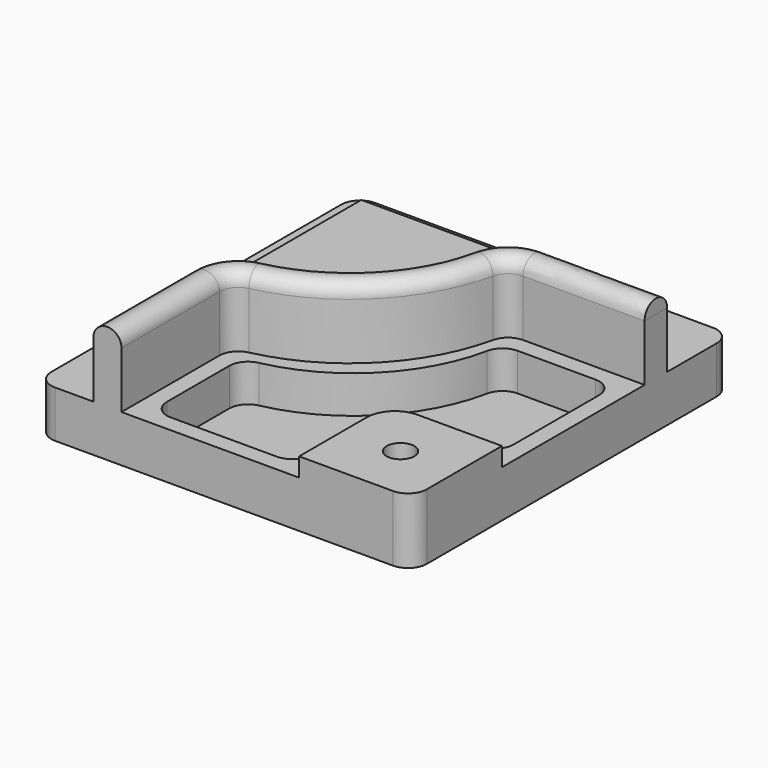
from build123d import *

# Parameters (mm, degrees)
F1_DEPTH        = 35
F2_DEPTH        = 25
F3_DEPTH        = 55
F4_DEPTH        = 25
F5_DEPTH        = 33
F6_DEPTH        = 5
F9_SIZE         = 4.5
F10_D           = 14.75
F10_CBORE_D     = 22.25
F10_CBORE_DEPTH = 14


with BuildPart() as f1:
    # F0 (on Top) → F1 (new body)
    with BuildSketch(Plane.XY):
        with BuildLine():
            Line((100, -96.5), (100, -46.5))
            Line((100, -46.5), (55, -46.5))
            ThreePointArc((55, -46.5), (44.393398, -50.893398), (40, -61.5))
            Line((40, -61.5), (40, -106.5))
            Line((40, -106.5), (90, -106.5))
            ThreePointArc((90, -106.5), (97.071068, -103.571068), (100, -96.5))
        make_face()
    extrude(amount=F1_DEPTH)

    # F0 (on Top) → F2 (join)
    with BuildSketch(Plane.XY):
        with BuildLine():
            Line((100, -46.5), (100, 48.5))
            Line((100, 48.5), (35.260832, 48.5))
            ThreePointArc((35.260832, 48.5), (29.00115, 46.298485), (25.497624, 40.663275))
            ThreePointArc((25.497624, 40.663275), (-0.104824, -5.979511), (-46.775973, -31.53022))
            ThreePointArc((-46.775973, -31.53022), (-52.418539, -35.031816), (-54.623526, -41.295822))
            Line((-54.623526, -41.295822), (-54.623526, -106.5))
            Line((-54.623526, -106.5), (40, -106.5))
            Line((40, -106.5), (40, -61.5))
            ThreePointArc((40, -61.5), (44.393398, -50.893398), (55, -46.5))
            Line((55, -46.5), (100, -46.5))
        make_face()
        with BuildLine():
            Line((31, -62.5), (31, -87.5))
            ThreePointArc((31, -87.5), (28.071068, -94.571068), (21, -97.5))
            Line((21, -97.5), (-35.623526, -97.5))
            ThreePointArc((-35.623526, -97.5), (-42.694594, -94.571068), (-45.623526, -87.5))
            Line((-45.623526, -87.5), (-45.623526, -46.002816))
            ThreePointArc((-45.623526, -46.002816), (-43.385729, -39.698199), (-37.673886, -36.215272))
            ThreePointArc((-37.673886, -36.215272), (6.161704, -12.434582), (29.746581, 31.506672))
            ThreePointArc((29.746581, 31.506672), (33.221258, 37.24812), (39.543175, 39.5))
            Line((39.543175, 39.5), (81, 39.5))
            ThreePointArc((81, 39.5), (88.071068, 36.571068), (91, 29.5))
            Line((91, 29.5), (91, -27.5))
            ThreePointArc((91, -27.5), (88.071068, -34.571068), (81, -37.5))
            Line((81, -37.5), (56, -37.5))
            ThreePointArc((56, -37.5), (38.32233, -44.82233), (31, -62.5))
        make_face(mode=Mode.SUBTRACT)
    extrude(amount=F2_DEPTH)

    # F0 (on Top) → F3 (join)
    with BuildSketch(Plane.XY):
        with BuildLine():
            Line((100, 48.5), (100, 63.5))
            Line((100, 63.5), (35.735586, 63.5))
            ThreePointArc((35.735586, 63.5), (20.232292, 58.112442), (11.41099, 44.27183))
            ThreePointArc((11.41099, 44.27183), (-10.73246, 4.608934), (-50.395356, -17.534515))
            ThreePointArc((-50.395356, -17.534515), (-64.235968, -26.355818), (-69.623526, -41.859112))
            Line((-69.623526, -41.859112), (-69.623526, -106.5))
            Line((-69.623526, -106.5), (-54.623526, -106.5))
            Line((-54.623526, -106.5), (-54.623526, -41.295822))
            ThreePointArc((-54.623526, -41.295822), (-52.418539, -35.031816), (-46.775973, -31.53022))
            ThreePointArc((-46.775973, -31.53022), (-0.104824, -5.979511), (25.497624, 40.663275))
            ThreePointArc((25.497624, 40.663275), (29.00115, 46.298485), (35.260832, 48.5))
            Line((35.260832, 48.5), (100, 48.5))
        make_face()
    extrude(amount=F3_DEPTH)

    # F0 (on Top) → F4 (join)
    with BuildSketch(Plane.XY):
        with BuildLine():
            Line((90, 106.5), (-90, 106.5))
            ThreePointArc((-90, 106.5), (-97.071068, 103.571068), (-100, 96.5))
            Line((-100, 96.5), (-100, -96.5))
            ThreePointArc((-100, -96.5), (-97.071068, -103.571068), (-90, -106.5))
            Line((-90, -106.5), (-69.623526, -106.5))
            Line((-69.623526, -106.5), (-69.623526, -41.859112))
            ThreePointArc((-69.623526, -41.859112), (-64.235968, -26.355818), (-50.395356, -17.534515))
            ThreePointArc((-50.395356, -17.534515), (-10.73246, 4.608934), (11.41099, 44.27183))
            ThreePointArc((11.41099, 44.27183), (20.232292, 58.112442), (35.735586, 63.5))
            Line((35.735586, 63.5), (100, 63.5))
            Line((100, 63.5), (100, 96.5))
            ThreePointArc((100, 96.5), (97.071068, 103.571068), (90, 106.5))
        make_face()
        with BuildLine():
            ThreePointArc((3.895179, 97.5), (-7.793942, 11.173118), (-91, -14.628397))
            Line((-91, -14.628397), (-91, 97.5))
            Line((-91, 97.5), (3.895179, 97.5))
        make_face(mode=Mode.SUBTRACT)
    extrude(amount=F4_DEPTH)

    # F0 (on Top) → F5 (join)
    with BuildSketch(Plane.XY):
        with BuildLine():
            Line((-91, 97.5), (-91, -14.628397))
            ThreePointArc((-91, -14.628397), (-7.793942, 11.173118), (3.895179, 97.5))
            Line((3.895179, 97.5), (-91, 97.5))
        make_face()
    extrude(amount=F5_DEPTH)

    # F0 (on Top) → F6 (join)
    with BuildSketch(Plane.XY):
        with BuildLine():
            ThreePointArc((21, -97.5), (28.071068, -94.571068), (31, -87.5))
            Line((31, -87.5), (31, -62.5))
            ThreePointArc((31, -62.5), (38.32233, -44.82233), (56, -37.5))
            Line((56, -37.5), (81, -37.5))
            ThreePointArc((81, -37.5), (88.071068, -34.571068), (91, -27.5))
            Line((91, -27.5), (91, 29.5))
            ThreePointArc((91, 29.5), (88.071068, 36.571068), (81, 39.5))
            Line((81, 39.5), (39.543175, 39.5))
            ThreePointArc((39.543175, 39.5), (33.221258, 37.24812), (29.746581, 31.506672))
            ThreePointArc((29.746581, 31.506672), (6.161704, -12.434582), (-37.673886, -36.215272))
            ThreePointArc((-37.673886, -36.215272), (-43.385729, -39.698199), (-45.623526, -46.002816))
            Line((-45.623526, -46.002816), (-45.623526, -87.5))
            ThreePointArc((-45.623526, -87.5), (-42.694594, -94.571068), (-35.623526, -97.5))
            Line((-35.623526, -97.5), (21, -97.5))
        make_face()
    extrude(amount=F6_DEPTH)

    # F8: sweep along a path in F8_path
    with BuildLine(Plane(origin=(-54.623526, -41.295822, 55), x_dir=(0, -1, 0), z_dir=(0, 0, -1))) as f8_path:
        Line((65.204178, 0), (0, 0))
        ThreePointArc((0, 0), (-6.264006, -2.204987), (-9.765602, -7.847553))
        ThreePointArc((-9.765602, -7.847553), (-35.31631, -54.518702), (-81.959096, -80.12115))
        ThreePointArc((-81.959096, -80.12115), (-87.594307, -83.624676), (-89.795822, -89.884358))
        Line((-89.795822, -89.884358), (-89.795822, -154.623526))
    # F7 (on face) → F8 (sweep)
    with BuildSketch(Plane.XZ.offset(106.5)):
        with BuildLine():
            ThreePointArc((-54.623526, 55), (-62.123526, 62.5), (-69.623526, 55))
            Line((-69.623526, 55), (-54.623526, 55))
        make_face()
    sweep(path=f8_path.line)

    # F9
    f9_edges = [f1.edges().sort_by_distance(p)[0] for p in [
        (-43.55241, 97.5, 33),
        (-91, 41.435802, 33),
        (-7.793942, 11.173118, 33),
    ]]
    chamfer(f9_edges, length=F9_SIZE)

    # F10 (through all)
    with Locations(Plane(origin=(0, 0, 0), x_dir=(1, 0, 0), z_dir=(0, 0, -1))):
        with Locations((70, 76.5)):
            CounterBoreHole(F10_D / 2, F10_CBORE_D / 2, F10_CBORE_DEPTH)


solid = f1.part
